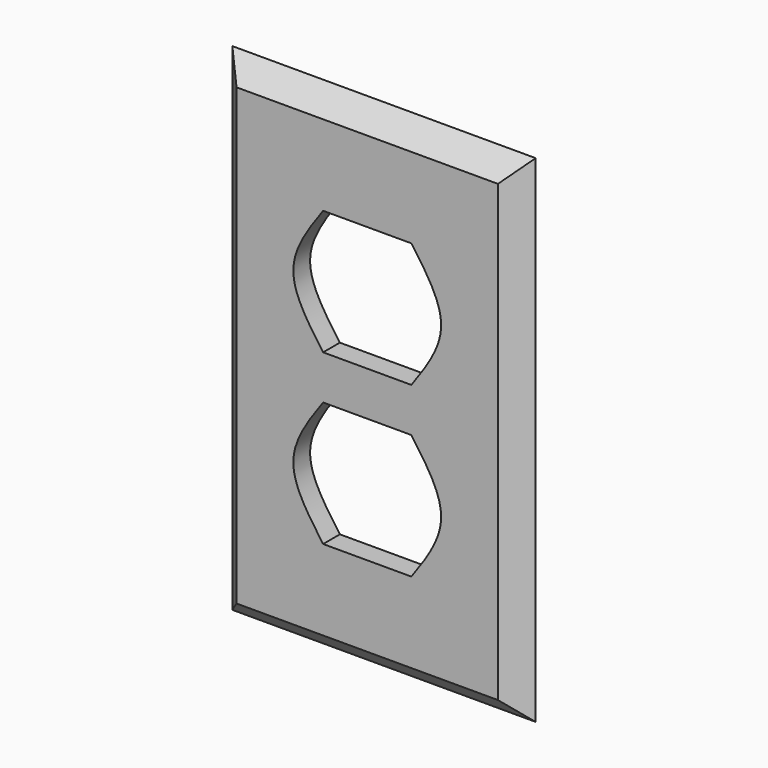
from build123d import *

# Parameters (mm, degrees)
F0_W     = 69.85
F0_H     = 114.3
F1_DEPTH = 4.826
F2_SIZE  = 4.82599


# Not quite as in the source:
# - a fillet or chamfer is up to 0.001 mm smaller than in the source, because OpenCascade refuses the exact size


with BuildPart() as f1:
    # F0 (on Front) → F1 (new body)
    with BuildSketch(Plane.XZ):
        Rectangle(F0_W, F0_H)
        with BuildLine():
            add(Edge.make_bspline(
                [(-10.16, -5.08), (-13.589, -9.8636666667), (-20.447, -19.431), (-13.589, -28.9983333333), (-10.16, -33.782)],
                knots=[0, 0, 0, 0, 0.5, 1, 1, 1, 1], degree=3))
            Line((-10.16, -5.08), (10.16, -5.08))
            add(Edge.make_bspline(
                [(10.16, -5.08), (13.589, -9.8636666667), (20.447, -19.431), (13.589, -28.9983333333), (10.16, -33.782)],
                knots=[0, 0, 0, 0, 0.5, 1, 1, 1, 1], degree=3))
            Line((10.16, -33.782), (-10.16, -33.782))
        make_face(mode=Mode.SUBTRACT)
        with BuildLine():
            add(Edge.make_bspline(
                [(-10.16, 33.782), (-13.589, 28.9983333333), (-20.447, 19.431), (-13.589, 9.8636666667), (-10.16, 5.08)],
                knots=[0, 0, 0, 0, 0.5, 1, 1, 1, 1], degree=3))
            Line((-10.16, 33.782), (10.16, 33.782))
            add(Edge.make_bspline(
                [(10.16, 33.782), (13.589, 28.9983333333), (20.447, 19.431), (13.589, 9.8636666667), (10.16, 5.08)],
                knots=[0, 0, 0, 0, 0.5, 1, 1, 1, 1], degree=3))
            Line((10.16, 5.08), (-10.16, 5.08))
        make_face(mode=Mode.SUBTRACT)
    extrude(amount=F1_DEPTH)

    # F2 (size 4.826 in the source; OpenCascade refuses exactly that, so slightly less here)
    f2_edges = [f1.edges().sort_by_distance(p)[0] for p in [
        (-34.925, -4.826, 0),
        (0, -4.826, 57.15),
        (34.925, -4.826, 0),
        (0, -4.826, -57.15),
    ]]
    chamfer(f2_edges, length=F2_SIZE)


solid = f1.part
